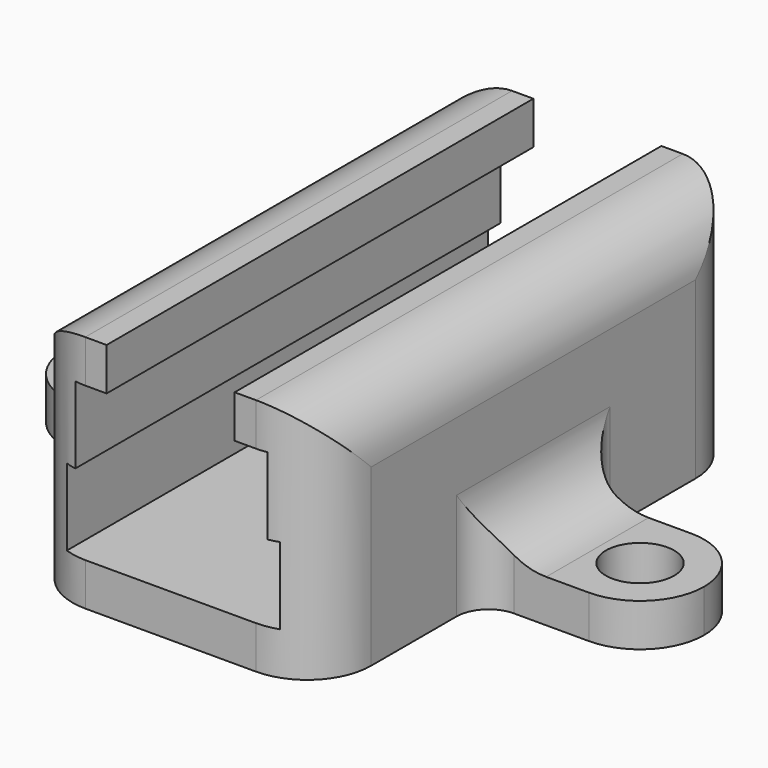
from build123d import *

# Parameters (mm, degrees)
F1_DEPTH    = 25
F2_R        = 1.6
F3_DEPTH    = 2
F4_F1_R     = 3
F4_T2_DEPTH = 17
F4_T4_DEPTH = 26.2
F4_T6_DEPTH = 40


# Not quite as in the source:
# - a fillet or chamfer that OpenCascade refuses, or shapes differently, is made with other operations: its cross-section is extruded or revolved along the edge and cut away or added


with BuildPart() as f1:
    # F0 (on Front) → F1 (new body)
    with BuildSketch(Plane.XZ):
        Polygon((0, 2), (0, 0), (7, 0), (7, 11.2), (3, 11.2), (3, 9.2), (4.5, 9.2), (4.5, 5.6), (5, 5.6), (5, 2), align=None)
    extrude(amount=F1_DEPTH)

    # F2 (on Top) → F3 (join)
    with BuildSketch(Plane.XY):
        with BuildLine():
            Line((15, -9.5), (8.5, -9.5))
            ThreePointArc((8.5, -9.5), (7.4393398282, -9.0606601718), (7, -8))
            Line((7, -8), (0, -8))
            Line((0, -8), (0, -9.5))
            Line((0, -9.5), (0, -15.5))
            Line((0, -15.5), (0, -17))
            Line((0, -17), (7, -17))
            ThreePointArc((7, -17), (7.4393398282, -15.9393398282), (8.5, -15.5))
            Line((8.5, -15.5), (15, -15.5))
            Line((15, -15.5), (15, -9.5))
        make_face()
        with Locations((12, -12.5)):
            Circle(F2_R, mode=Mode.SUBTRACT)
    extrude(amount=F3_DEPTH)

    # F4: fillet of radius 3 on 6 edges, made by hand

    # F4_f1
    f4_f1_edges = [f1.edges().sort_by_distance(p)[0] for p in [
        (7, -12.5, 2),
    ]]
    fillet(f4_f1_edges, radius=F4_F1_R)

    # F4_s3 → F4_t2 (cut)
    with BuildSketch(Plane.XY.offset(-7.5)):
        with BuildLine():
            ThreePointArc((15, -12.5), (14.1213203436, -14.6213203436), (12, -15.5))
            Line((12, -15.5), (12, -15.56))
            Line((12, -15.56), (15.06, -15.56))
            Line((15.06, -15.56), (15.06, -12.5))
            Line((15.06, -12.5), (15, -12.5))
        make_face()
        with BuildLine():
            ThreePointArc((12, -9.5), (14.1213203436, -10.3786796564), (15, -12.5))
            Line((15, -12.5), (15.06, -12.5))
            Line((15.06, -12.5), (15.06, -9.44))
            Line((15.06, -9.44), (12, -9.44))
            Line((12, -9.44), (12, -9.5))
        make_face()
    extrude(amount=F4_T2_DEPTH, mode=Mode.SUBTRACT)

    # F4_s5 → F4_t4 (cut)
    with BuildSketch(Plane.XY.offset(-7.5)):
        with BuildLine():
            ThreePointArc((7, -22), (6.1213203436, -24.1213203436), (4, -25))
            Line((4, -25), (4, -25.06))
            Line((4, -25.06), (7.06, -25.06))
            Line((7.06, -25.06), (7.06, -22))
            Line((7.06, -22), (7, -22))
        make_face()
        with BuildLine():
            ThreePointArc((7, -3), (6.1213203436, -0.8786796564), (4, 0))
            Line((4, 0), (4, 0.06))
            Line((4, 0.06), (7.06, 0.06))
            Line((7.06, 0.06), (7.06, -3))
            Line((7.06, -3), (7, -3))
        make_face()
    extrude(amount=F4_T4_DEPTH, mode=Mode.SUBTRACT)

    # F4_s7 → F4_t6 (cut)
    with BuildSketch(Plane.XZ.offset(-7.5)):
        with BuildLine():
            ThreePointArc((7, 8.2), (6.1213203436, 10.3213203436), (4, 11.2))
            Line((4, 11.2), (4, 11.26))
            Line((4, 11.26), (7.06, 11.26))
            Line((7.06, 11.26), (7.06, 8.2))
            Line((7.06, 8.2), (7, 8.2))
        make_face()
    extrude(amount=F4_T6_DEPTH, mode=Mode.SUBTRACT)

    # F5: F1 across face


with BuildPart() as f1_1:
    add(f1.part)
    add(f1.part.mirror(Plane(origin=(0, -12.5, 1), x_dir=(0, -1, 0), z_dir=(-1, 0, 0))))


solid = f1_1.part
